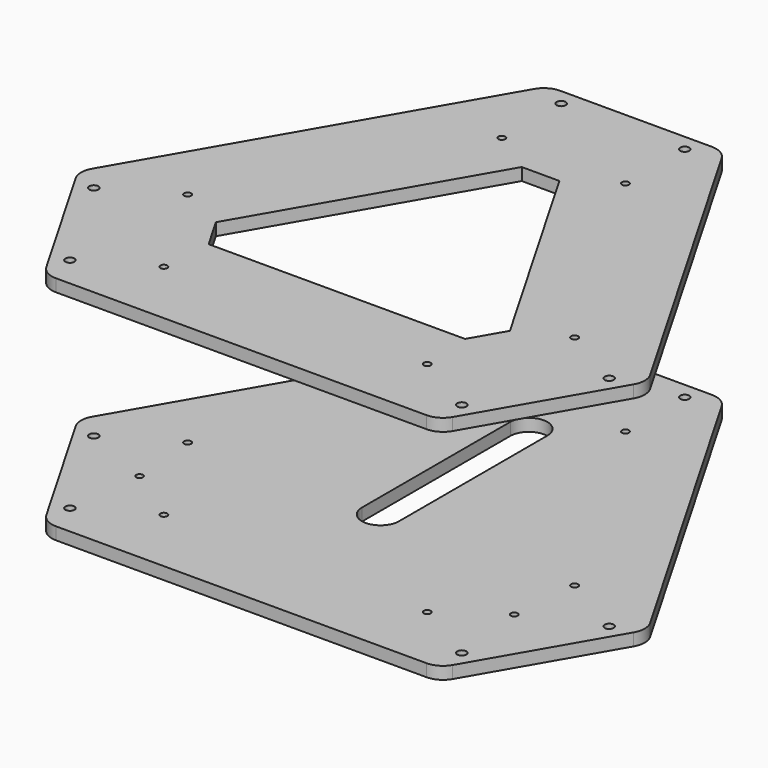
from build123d import *

# Parameters (mm, degrees)
F0_R     = 2.2
F0_R_2   = 1.7
F1_DEPTH = 6
F3_R     = 2.2
F3_R_2   = 1.7
F3_R_3   = 1.65
F4_DEPTH = 6
F5_R     = 10
F5_2_R   = 10


# Not quite as in the source:
# - a feature names something its author has since deleted; it is built from what else it names


with BuildPart() as f1:
    # F0 (on Top) → F1 (new body)
    with BuildSketch(Plane.XY):
        Polygon((-42.617, 135.14210956), (-138.345, -30.6636501469), (-95.728, -104.4784594131), (95.728, -104.4784594131), (138.345, -30.6636501469), (42.617, 135.14210956), align=None)
        with Locations((-95.1082967697, -89.5518168935)):
            Circle(F0_R, mode=Mode.SUBTRACT)
        with Locations((-63.9313822335, -71.5518168935)):
            Circle(F0_R_2, mode=Mode.SUBTRACT)
        with Locations((-125.1082967697, -37.5902926665)):
            Circle(F0_R, mode=Mode.SUBTRACT)
        with Locations((-93.9313822335, -19.5902926665)):
            Circle(F0_R_2, mode=Mode.SUBTRACT)
        with Locations((63.9313822335, -71.5518168935)):
            Circle(F0_R_2, mode=Mode.SUBTRACT)
        with Locations((95.1082967697, -89.5518168935)):
            Circle(F0_R, mode=Mode.SUBTRACT)
        Polygon((71.372368774, -30.6636501469), (62.241684387, -46.4784594131), (-62.241684387, -46.4784594131), (-71.372368774, -30.6636501469), (-9.130684387, 77.14210956), (9.130684387, 77.14210956), align=None, mode=Mode.SUBTRACT)
        with Locations((93.9313822335, -19.5902926665)):
            Circle(F0_R_2, mode=Mode.SUBTRACT)
        with Locations((125.1082967697, -37.5902926665)):
            Circle(F0_R, mode=Mode.SUBTRACT)
        with Locations((-30, 91.14210956)):
            Circle(F0_R_2, mode=Mode.SUBTRACT)
        with Locations((-30, 127.14210956)):
            Circle(F0_R, mode=Mode.SUBTRACT)
        with Locations((30, 91.14210956)):
            Circle(F0_R_2, mode=Mode.SUBTRACT)
        with Locations((30, 127.14210956)):
            Circle(F0_R, mode=Mode.SUBTRACT)
    extrude(amount=F1_DEPTH)

    # F5
    f5_edges = [f1.edges().sort_by_distance(p)[0] for p in [
        (95.728, -104.478459, 3),
        (138.345, -30.66365, 3),
        (-95.728, -104.478459, 3),
        (-138.345, -30.66365, 3),
        (-42.617, 135.14211, 3),
        (42.617, 135.14211, 3),
    ]]
    fillet(f5_edges, radius=F5_R)


with BuildPart() as f4:
    # F3 (on offset) → F4 (new body)
    with BuildSketch(Plane(origin=(0, 0, -100), x_dir=(1, 0, 0), z_dir=(0, 0, -1))):
        Polygon((95.728, 104.4784594131), (-95.728, 104.4784594131), (-138.345, 30.6636501469), (-42.617, -135.14210956), (42.617, -135.14210956), (138.345, 30.6636501469), align=None)
        with Locations((-30, -127.14210956)):
            Circle(F3_R, mode=Mode.SUBTRACT)
        with Locations((-30, -91.14210956)):
            Circle(F3_R_2, mode=Mode.SUBTRACT)
        with Locations((0, -105)):
            Circle(F3_R_3, mode=Mode.SUBTRACT)
        with BuildLine():
            Line((-9, -70), (-9, 20))
            ThreePointArc((-9, 20), (0, 29), (9, 20))
            Line((9, 20), (9, -70))
            ThreePointArc((9, -70), (0, -79), (-9, -70))
        make_face(mode=Mode.SUBTRACT)
        with Locations((30, -127.14210956)):
            Circle(F3_R, mode=Mode.SUBTRACT)
        with Locations((30, -91.14210956)):
            Circle(F3_R_2, mode=Mode.SUBTRACT)
        with Locations((-125.1082967697, 37.5902926665)):
            Circle(F3_R, mode=Mode.SUBTRACT)
        with Locations((-93.9313822335, 19.5902926665)):
            Circle(F3_R_2, mode=Mode.SUBTRACT)
        with Locations((-90.9326673974, 52.5)):
            Circle(F3_R_3, mode=Mode.SUBTRACT)
        with Locations((-95.1082967697, 89.5518168935)):
            Circle(F3_R, mode=Mode.SUBTRACT)
        with Locations((-63.9313822335, 71.5518168935)):
            Circle(F3_R_2, mode=Mode.SUBTRACT)
        with Locations((93.9313822335, 19.5902926665)):
            Circle(F3_R_2, mode=Mode.SUBTRACT)
        with Locations((125.1082967697, 37.5902926665)):
            Circle(F3_R, mode=Mode.SUBTRACT)
        with Locations((63.9313822335, 71.5518168935)):
            Circle(F3_R_2, mode=Mode.SUBTRACT)
        with Locations((90.9326673974, 52.5)):
            Circle(F3_R_3, mode=Mode.SUBTRACT)
        with Locations((95.1082967697, 89.5518168935)):
            Circle(F3_R, mode=Mode.SUBTRACT)
    extrude(amount=F4_DEPTH)

    # F5#2
    f5_2_edges = [f4.edges().sort_by_distance(p)[0] for p in [
        (-42.617, 135.14211, -103),
        (42.617, 135.14211, -103),
        (138.345, -30.66365, -103),
        (95.728, -104.478459, -103),
        (-95.728, -104.478459, -103),
        (-138.345, -30.66365, -103),
    ]]
    fillet(f5_2_edges, radius=F5_2_R)


solid = Compound([f1.part, f4.part])
